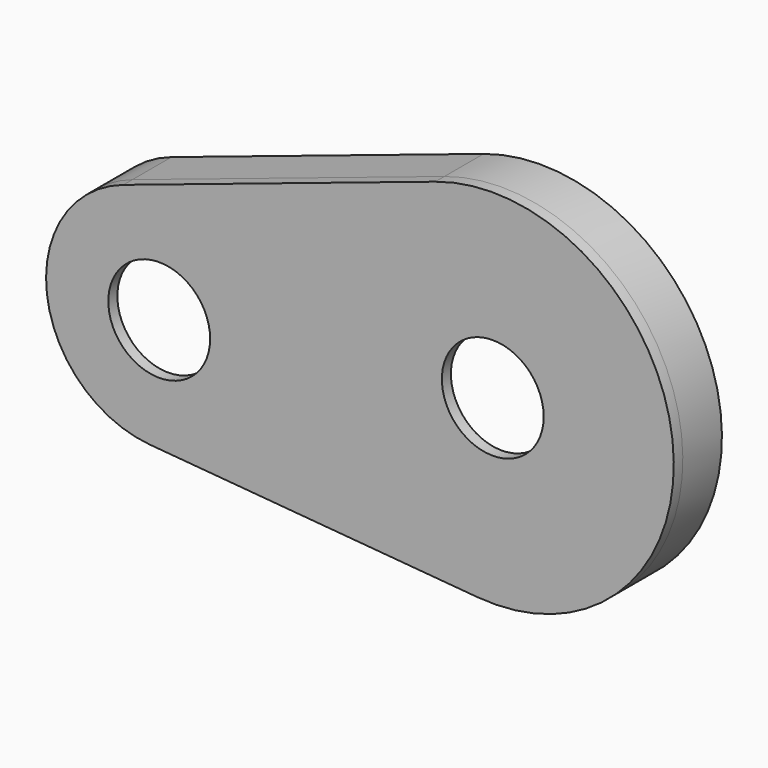
from build123d import *
from build123d import SkipClean  # not in build123d's __all__

# Parameters (mm, degrees)
F0_R     = 14.2875
F1_DEPTH = 3.175
F3_DEPTH = 13.716


# Not quite as in the source:
# - a feature names something its author has since deleted; it is built from what else it names


with BuildPart() as f1:
    # F0 (on Front) → F1 (new body)
    with BuildSketch(Plane.XZ):
        with BuildLine():
            Line((-96.2781986811, -42.8291897772), (-4.2862845567, -50.6188479195))
            ThreePointArc((-4.2862845567, -50.6188479195), (50.4406573252, 6.0315908845), (-16.1005722699, 48.1810291773))
            Line((-16.1005722699, 48.1810291773), (-103.6621285019, 18.9207334083))
            ThreePointArc((-103.6621285019, 18.9207334083), (-125.3487825032, -11.3685027389), (-103.3274855148, -41.4153206587))
            ThreePointArc((-103.3274855148, -41.4153206587), (-99.8429919119, -42.3224346764), (-96.2781986811, -42.8291897772))
        make_face()
        with BuildLine():
            Line((-102.655842735, 15.9094190847), (-15.0942865031, 45.1697148537))
            ThreePointArc((-15.0942865031, 45.1697148537), (47.2881162424, 5.6546164542), (-4.0183917719, -47.4551699245))
            Line((-4.0183917719, -47.4551699245), (-96.0103058963, -39.6655117822))
            ThreePointArc((-96.0103058963, -39.6655117822), (-121.9721405786, -14.5851797), (-102.655842735, 15.9094190847))
        make_face(mode=Mode.SUBTRACT)
        with BuildLine():
            ThreePointArc((-4.0183917719, -47.4551699245), (47.2881162424, 5.6546164542), (-15.0942865031, 45.1697148537))
            Line((-15.0942865031, 45.1697148537), (-102.655842735, 15.9094190847))
            ThreePointArc((-102.655842735, 15.9094190847), (-121.9721405786, -14.5851797), (-96.0103058963, -39.6655117822))
            Line((-96.0103058963, -39.6655117822), (-4.0183917719, -47.4551699245))
        make_face()
        with Locations((-93.5992708332, -11.1924098275)):
            Circle(F0_R, mode=Mode.SUBTRACT)
        Circle(F0_R, mode=Mode.SUBTRACT)
    extrude(amount=F1_DEPTH)

    # F2 (on face) → F3 (join)
    with BuildSketch(Plane(origin=(0, 0, 0), x_dir=(-1, 0, 0), z_dir=(0, 1, 0))):
        with BuildLine():
            ThreePointArc((96.2781986811, -42.8291897772), (125.1246816615, -14.9621541303), (103.6621285019, 18.9207334083))
            Line((103.6621285019, 18.9207334083), (16.1005722699, 48.1810291773))
            ThreePointArc((16.1005722699, 48.1810291773), (-50.4406573252, 6.0315908845), (4.2862845567, -50.6188479195))
            Line((4.2862845567, -50.6188479195), (96.2781986811, -42.8291897772))
        make_face()
        with BuildLine():
            Line((15.0942865031, 45.1697148537), (102.655842735, 15.9094190847))
            ThreePointArc((102.655842735, 15.9094190847), (121.9721405786, -14.5851797), (96.0103058963, -39.6655117822))
            Line((96.0103058963, -39.6655117822), (4.0183917719, -47.4551699245))
            ThreePointArc((4.0183917719, -47.4551699245), (-47.2881162424, 5.6546164542), (15.0942865031, 45.1697148537))
        make_face(mode=Mode.SUBTRACT)
    with SkipClean():  # cleaning this boolean's faces spoils the solid; the shape is the same uncleaned
        extrude(amount=F3_DEPTH)


solid = f1.part
